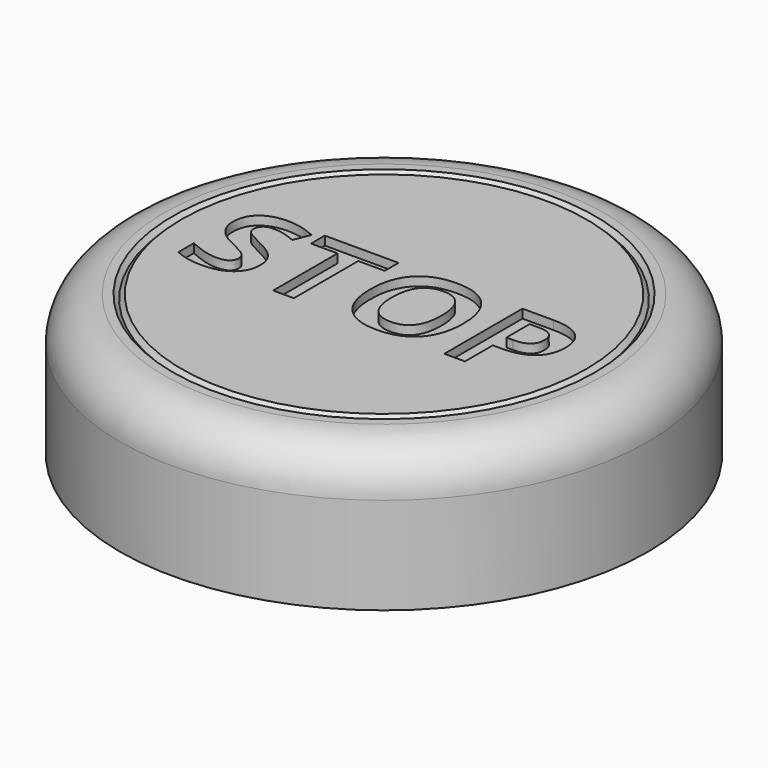
from build123d import *

# Parameters (mm, degrees)
F0_R         = 15
F1_DEPTH     = 8
F2_R         = 12
F2_R_2       = 11.5
F3_DEPTH     = 0.5
F3_TAPER     = 45
F4_R         = 2.5
F5_TEXT_SIZE = 7.7712342906
F6_DEPTH     = 0.5
F7_R         = 1.5
F8_DEPTH     = 0.15


# Not quite as in the source:
# - Text() gives the source's letters only with a copy of the font that has no kerning and outlines rounded to 1/6400 em; it was checked with that copy


with BuildPart() as f1:
    # F0 (on Top) → F1 (new body)
    with BuildSketch(Plane.XY):
        Circle(F0_R)
    extrude(amount=F1_DEPTH)

    # F2 (on face) → F3 (cut)
    with BuildSketch(Plane.XY.offset(8)):
        Circle(F2_R)
        Circle(F2_R_2, mode=Mode.SUBTRACT)
    extrude(amount=-F3_DEPTH, taper=F3_TAPER, mode=Mode.SUBTRACT)

    # F4
    f4_edges = [f1.edges().sort_by_distance(p)[0] for p in [
        (-15, 0, 8),
    ]]
    fillet(f4_edges, radius=F4_R)

    # F5 (on face) → F6 (cut)
    with BuildSketch(Plane.XY.offset(8)):
        with Locations((-10, -2.7976443446)):
            Text('STOP', F5_TEXT_SIZE, font='Open Sans', font_style=FontStyle.BOLD, text_align=(TextAlign.LEFT, TextAlign.BOTTOM))
    extrude(amount=-F6_DEPTH, mode=Mode.SUBTRACT)

    # F7 (on face) → F8 (cut)
    with BuildSketch(Plane(origin=(0, 0, 0), x_dir=(1, 0, 0), z_dir=(0, 0, -1))):
        with Locations((0, -8)):
            Circle(F7_R)
        with Locations((6.9282032303, 4)):
            Circle(F7_R)
        with Locations((-6.9282032303, 4)):
            Circle(F7_R)
    extrude(amount=-F8_DEPTH, mode=Mode.SUBTRACT)


solid = f1.part
